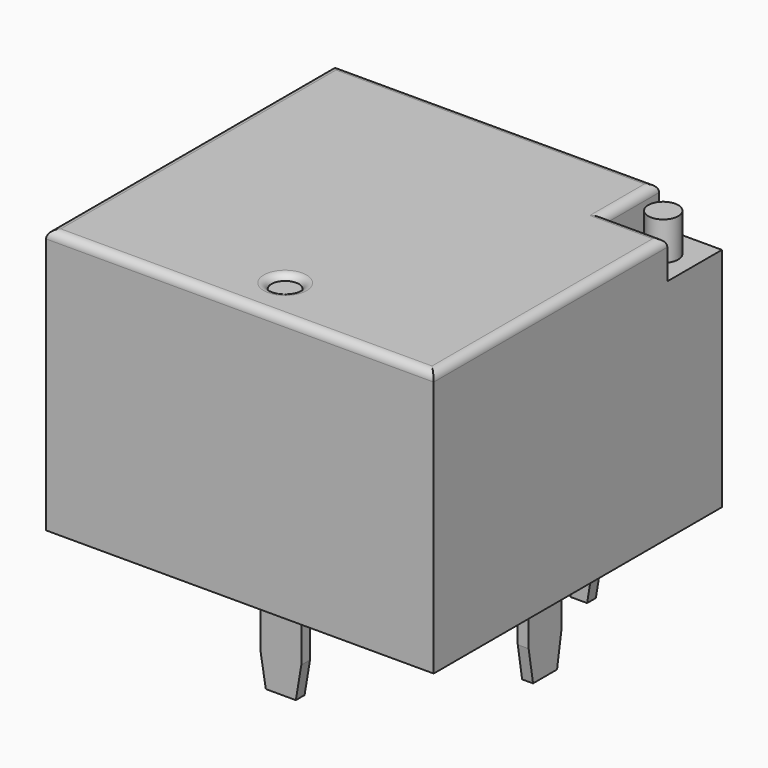
from build123d import *

# Parameters (mm, degrees)
F1_W         = 14.2
F1_H         = 13.2
F2_DEPTH     = 9.7
F0_W         = 0.4
F0_H         = 1.5
F3_DEPTH     = 3.5
F0_W_2       = 1.5
F0_H_2       = 0.4
F0_W_3       = 1
F4_W         = 2.3
F4_H         = 2.5
F4_R         = 0.55
F5_DEPTH     = 1.4
F4_R_2       = 0.5
F6_DEPTH     = 0.2
F7_T1_DEPTH  = 3.25
F7_T3_DEPTH  = 13.4
F7_T5_DEPTH  = 3.05
F7_T7_DEPTH  = 14.7
F7_T9_DEPTH  = 12.2
F7_T11_DEPTH = 15.7
F7_T19_DEPTH = 3.25
F7_T23_DEPTH = 3.05
F8_SIZE2     = 1.2
F8_SIZE      = 0.2
F8_2_SIZE2   = 1.2
F8_2_SIZE    = 0.2
F8_3_SIZE2   = 1.2
F8_3_SIZE    = 0.2
F8_4_SIZE2   = 1.2
F8_4_SIZE    = 0.2
F8_5_SIZE2   = 1.2
F8_5_SIZE    = 0.2


# Not quite as in the source:
# - a fillet or chamfer that OpenCascade refuses, or shapes differently, is made with other operations: its cross-section is extruded or revolved along the edge and cut away or added


with BuildPart() as f2:
    # F1 (on Top) → F2 (new body)
    with BuildSketch(Plane.XY):
        with Locations((-0.3, -0.5)):
            Rectangle(F1_W, F1_H)
    extrude(amount=F2_DEPTH)

    # F4 (on face) → F5 (cut)
    with BuildSketch(Plane.XY.offset(9.7)):
        with Locations((5.65, 4.85)):
            Rectangle(F4_W, F4_H)
        with Locations((5.65, 4.85)):
            Circle(F4_R, mode=Mode.SUBTRACT)
    extrude(amount=-F5_DEPTH, mode=Mode.SUBTRACT)

    # F4 (on face) → F6 (cut)
    with BuildSketch(Plane.XY.offset(9.7)):
        with Locations((0, -5.4)):
            Circle(F4_R_2)
    extrude(amount=-F6_DEPTH, mode=Mode.SUBTRACT)

    # F7: fillet of radius 0.3 on 7 edges, made by hand

    # F7_s2 → F7_t1 (cut)
    with BuildSketch(Plane.XZ.offset(-6.85)):
        with BuildLine():
            ThreePointArc((4.2, 9.7), (4.4121320344, 9.6121320344), (4.5, 9.4))
            Line((4.5, 9.4), (4.5, 9.7))
            Line((4.5, 9.7), (4.2, 9.7))
        make_face()
    extrude(amount=F7_T1_DEPTH, mode=Mode.SUBTRACT)

    # F7_s4 → F7_t3 (cut)
    with BuildSketch(Plane.YZ.offset(-8.15)):
        with BuildLine():
            ThreePointArc((6.1, 9.4), (6.0121320344, 9.6121320344), (5.8, 9.7))
            Line((5.8, 9.7), (6.1, 9.7))
            Line((6.1, 9.7), (6.1, 9.4))
        make_face()
    extrude(amount=F7_T3_DEPTH, mode=Mode.SUBTRACT)

    # F7_s6 → F7_t5 (cut)
    with BuildSketch(Plane.YZ.offset(4.5)):
        with BuildLine():
            ThreePointArc((3.3, 9.7), (3.5121320344, 9.6121320344), (3.6, 9.4))
            Line((3.6, 9.4), (3.6, 9.7))
            Line((3.6, 9.7), (3.3, 9.7))
        make_face()
    extrude(amount=F7_T5_DEPTH, mode=Mode.SUBTRACT)

    # F7_s8 → F7_t7 (cut)
    with BuildSketch(Plane.XZ.offset(-6.85)):
        with BuildLine():
            ThreePointArc((-7.4, 9.4), (-7.3121320344, 9.6121320344), (-7.1, 9.7))
            Line((-7.1, 9.7), (-7.4, 9.7))
            Line((-7.4, 9.7), (-7.4, 9.4))
        make_face()
    extrude(amount=F7_T7_DEPTH, mode=Mode.SUBTRACT)

    # F7_s10 → F7_t9 (cut)
    with BuildSketch(Plane.XZ.offset(-4.35)):
        with BuildLine():
            ThreePointArc((6.5, 9.7), (6.7121320344, 9.6121320344), (6.8, 9.4))
            Line((6.8, 9.4), (6.8, 9.7))
            Line((6.8, 9.7), (6.5, 9.7))
        make_face()
    extrude(amount=F7_T9_DEPTH, mode=Mode.SUBTRACT)

    # F7_s12 → F7_t11 (cut)
    with BuildSketch(Plane.YZ.offset(-8.15)):
        with BuildLine():
            ThreePointArc((-6.8, 9.7), (-7.0121320344, 9.6121320344), (-7.1, 9.4))
            Line((-7.1, 9.4), (-7.1, 9.7))
            Line((-7.1, 9.7), (-6.8, 9.7))
        make_face()
    extrude(amount=F7_T11_DEPTH, mode=Mode.SUBTRACT)

    # F7_s13 → F7_t14 (revolve, cut)
    with BuildSketch(Plane.XZ.offset(5.4)):
        with BuildLine():
            ThreePointArc((0.7828427125, 9.7), (0.6096376317, 9.6449489743), (0.5, 9.5))
            Line((0.5, 9.5), (0.5, 9.7))
            Line((0.5, 9.7), (0.7828427125, 9.7))
        make_face()
    revolve(axis=Axis((0, -5.4, 9.7), (0, 0, 1)), mode=Mode.SUBTRACT)


with BuildPart() as f3:
    # F0 (on Top) → F3 (new body)
    with BuildSketch(Plane.XY):
        with Locations((-5.7, 0)):
            Rectangle(F0_W, F0_H)
    extrude(amount=-F3_DEPTH)

    # F8
    f8_edges = [f3.edges().sort_by_distance(p)[0] for p in [
        (-5.7, -0.75, -3.5),
        (-5.7, 0.75, -3.5),
    ]]
    f8_side = f3.faces().sort_by_distance((-5.7, 0, -3.5))[0]
    chamfer(f8_edges, length=F8_SIZE, length2=F8_SIZE2, reference=f8_side)


with BuildPart() as f3b:
    # F0 (on Top) → F3, piece 2 (new body)
    with BuildSketch(Plane.XY):
        with Locations((5, 0)):
            Rectangle(F0_W, F0_H)
    extrude(amount=-F3_DEPTH)

    # F8#5
    f8_5_edges = [f3b.edges().sort_by_distance(p)[0] for p in [
        (5, -0.75, -3.5),
        (5, 0.75, -3.5),
    ]]
    f8_5_side = f3b.faces().sort_by_distance((5, 0, -3.5))[0]
    chamfer(f8_5_edges, length=F8_5_SIZE, length2=F8_5_SIZE2, reference=f8_5_side)


with BuildPart() as f3c:
    # F0 (on Top) → F3, piece 3 (new body)
    with BuildSketch(Plane.XY):
        with Locations((0, -5.4)):
            Rectangle(F0_W_2, F0_H_2)
    extrude(amount=-F3_DEPTH)

    # F8#2
    f8_2_edges = [f3c.edges().sort_by_distance(p)[0] for p in [
        (0.75, -5.4, -3.5),
        (-0.75, -5.4, -3.5),
    ]]
    f8_2_side = f3c.faces().sort_by_distance((0, -5.4, -3.5))[0]
    chamfer(f8_2_edges, length=F8_2_SIZE, length2=F8_2_SIZE2, reference=f8_2_side)


with BuildPart() as f3d:
    # F0 (on Top) → F3, piece 4 (new body)
    with BuildSketch(Plane.XY):
        with Locations((-3, 4.5)):
            Rectangle(F0_W_3, F0_H_2)
    extrude(amount=-F3_DEPTH)

    # F8#3
    f8_3_edges = [f3d.edges().sort_by_distance(p)[0] for p in [
        (-2.5, 4.5, -3.5),
        (-3.5, 4.5, -3.5),
    ]]
    f8_3_side = f3d.faces().sort_by_distance((-3, 4.5, -3.5))[0]
    chamfer(f8_3_edges, length=F8_3_SIZE, length2=F8_3_SIZE2, reference=f8_3_side)


with BuildPart() as f3e:
    # F0 (on Top) → F3, piece 5 (new body)
    with BuildSketch(Plane.XY):
        with Locations((3, 4.5)):
            Rectangle(F0_W_3, F0_H_2)
    extrude(amount=-F3_DEPTH)

    # F8#4
    f8_4_edges = [f3e.edges().sort_by_distance(p)[0] for p in [
        (2.5, 4.5, -3.5),
        (3.5, 4.5, -3.5),
    ]]
    f8_4_side = f3e.faces().sort_by_distance((3, 4.5, -3.5))[0]
    chamfer(f8_4_edges, length=F8_4_SIZE, length2=F8_4_SIZE2, reference=f8_4_side)


with BuildPart() as f7_tool17:
    # F7_s18 → F7_t19 (new body)
    with BuildSketch(Plane.XZ.offset(-6.1)):
        with BuildLine():
            ThreePointArc((4.2, 9.7), (4.4121320344, 9.6121320344), (4.5, 9.4))
            Line((4.5, 9.4), (4.5, 9.7))
            Line((4.5, 9.7), (4.2, 9.7))
        make_face()
    extrude(amount=F7_T19_DEPTH)

    split(bisect_by=Plane.XZ.offset(-3.6), keep=Keep.TOP)


with BuildPart() as f7_tool21:
    # F7_s22 → F7_t23 (new body)
    with BuildSketch(Plane.YZ.offset(3.75)):
        with BuildLine():
            ThreePointArc((3.3, 9.7), (3.5121320344, 9.6121320344), (3.6, 9.4))
            Line((3.6, 9.4), (3.6, 9.7))
            Line((3.6, 9.7), (3.3, 9.7))
        make_face()
    extrude(amount=F7_T23_DEPTH)

    split(bisect_by=Plane.YZ.offset(4.5), keep=Keep.BOTTOM)


with BuildPart() as f7_tool17_1:
    add(f7_tool17.part)

    # F7_t25: intersect F7_tool21
    add(f7_tool21.part, mode=Mode.INTERSECT)


with BuildPart() as f2_1:
    add(f2.part)

    # F7_t15: cut F7_tool17
    add(f7_tool17_1.part, mode=Mode.SUBTRACT)


solid = Compound([f3.part, f3b.part, f3c.part, f3d.part, f3e.part, f2_1.part])
